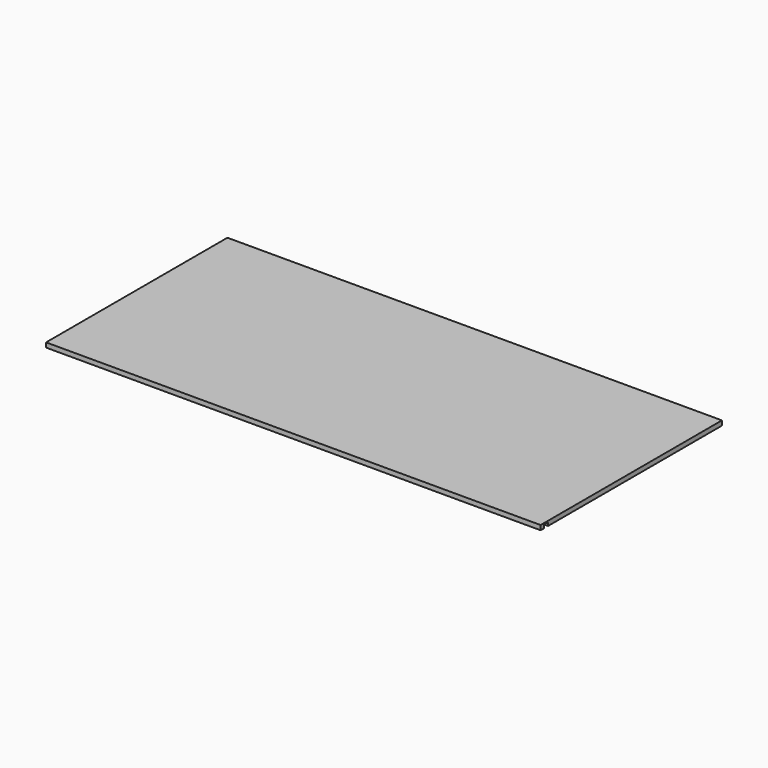
from build123d import *

# Parameters (mm, degrees)
F0_W     = 1920
F0_H     = 880
F1_DEPTH = 9
F2_W     = 1920
F2_H     = 20
F3_DEPTH = 13


with BuildPart() as f1:
    # F0 (on Top) → F1 (new body, symmetric)
    with BuildSketch(Plane.XY):
        Rectangle(F0_W, F0_H)
    extrude(amount=F1_DEPTH, both=True)

    # F2 (on face) → F3 (cut)
    with BuildSketch(Plane(origin=(0, 0, -9), x_dir=(1, 0, 0), z_dir=(0, 0, -1))):
        with Locations((0, 414)):
            Rectangle(F2_W, F2_H)
    extrude(amount=-F3_DEPTH, mode=Mode.SUBTRACT)


solid = f1.part
